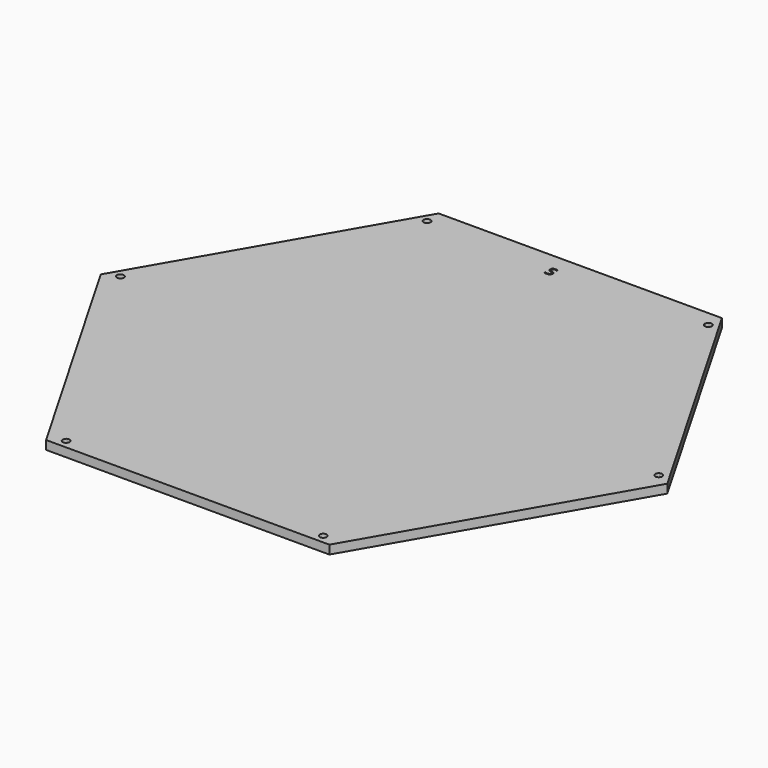
from build123d import *

# Parameters (mm, degrees)
F1_DEPTH     = 5
F3_DEPTH     = 25
F4_TEXT_SIZE = 8.1927412086
F5_DEPTH     = 25


# Not quite as in the source:
# - Text() gives the source's letters only with a copy of the font that has no kerning and outlines rounded to 1/6400 em; it was checked with that copy


with BuildPart() as f1:
    # F0 (on Top) → F1 (new body)
    with BuildSketch(Plane.XY):
        Polygon((-162, 140.2961154131), (-81, 0), (81, 0), (162, 140.2961154131), (81, 280.5922308262), (-81, 280.5922308262), align=None)
    extrude(amount=F1_DEPTH)

    # F2 (on face) → F3 (cut)
    with BuildSketch(Plane.XY.offset(5)):
        with BuildLine():
            Line((-78.4226497308, 271.5922308262), (-80.4226497308, 271.5922308262))
            Line((-80.4226497308, 271.5922308262), (-81.4226497308, 269.8601800186))
            ThreePointArc((-81.4226497308, 269.8601800186), (-79.4226497308, 269.8601800186), (-78.4226497308, 271.5922308262))
        make_face()
        with BuildLine():
            Line((-79.4226497308, 273.3242816337), (-80.4226497308, 271.5922308262))
            Line((-80.4226497308, 271.5922308262), (-78.4226497308, 271.5922308262))
            ThreePointArc((-78.4226497308, 271.5922308262), (-78.6905989232, 272.5922308262), (-79.4226497308, 273.3242816337))
        make_face()
        with BuildLine():
            Line((-81.4226497308, 269.8601800186), (-80.4226497308, 271.5922308262))
            Line((-80.4226497308, 271.5922308262), (-79.4226497308, 273.3242816337))
            ThreePointArc((-79.4226497308, 273.3242816337), (-82.1547005384, 272.5922308262), (-81.4226497308, 269.8601800186))
        make_face()
        with BuildLine():
            Line((79.4226497308, 273.3242816337), (80.4226497308, 271.5922308262))
            Line((80.4226497308, 271.5922308262), (81.4226497308, 269.8601800186))
            ThreePointArc((81.4226497308, 269.8601800186), (82.1547005384, 270.5922308262), (82.4226497308, 271.5922308262))
            ThreePointArc((82.4226497308, 271.5922308262), (81.4226497308, 273.3242816337), (79.4226497308, 273.3242816337))
        make_face()
        with BuildLine():
            ThreePointArc((79.4226497308, 273.3242816337), (78.6905989232, 272.5922308262), (78.4226497308, 271.5922308262))
            Line((78.4226497308, 271.5922308262), (80.4226497308, 271.5922308262))
            Line((80.4226497308, 271.5922308262), (79.4226497308, 273.3242816337))
        make_face()
        with BuildLine():
            Line((80.4226497308, 271.5922308262), (78.4226497308, 271.5922308262))
            ThreePointArc((78.4226497308, 271.5922308262), (79.4226497308, 269.8601800186), (81.4226497308, 269.8601800186))
            Line((81.4226497308, 269.8601800186), (80.4226497308, 271.5922308262))
        make_face()
        with BuildLine():
            ThreePointArc((155.9170962313, 144.2961154131), (154.9170962313, 146.0281662206), (152.9170962313, 146.0281662206))
            Line((152.9170962313, 146.0281662206), (153.9170962313, 144.2961154131))
            Line((153.9170962313, 144.2961154131), (154.9170962313, 142.5640646055))
            ThreePointArc((154.9170962313, 142.5640646055), (155.6491470389, 143.2961154131), (155.9170962313, 144.2961154131))
        make_face()
        with BuildLine():
            Line((154.9170962313, 142.5640646055), (153.9170962313, 144.2961154131))
            Line((153.9170962313, 144.2961154131), (152.9170962313, 142.5640646055))
            ThreePointArc((152.9170962313, 142.5640646055), (153.9170962313, 142.2961154131), (154.9170962313, 142.5640646055))
        make_face()
        with BuildLine():
            Line((153.9170962313, 144.2961154131), (152.9170962313, 146.0281662206))
            ThreePointArc((152.9170962313, 146.0281662206), (151.9170962313, 144.2961154131), (152.9170962313, 142.5640646055))
            Line((152.9170962313, 142.5640646055), (153.9170962313, 144.2961154131))
        make_face()
        with BuildLine():
            Line((73.494446436, 4.9999998882), (74.494446436, 6.7320506958))
            ThreePointArc((74.494446436, 6.7320506958), (72.494446436, 6.7320506958), (71.494446436, 4.9999998882))
            Line((71.494446436, 4.9999998882), (73.494446436, 4.9999998882))
        make_face()
        with BuildLine():
            ThreePointArc((75.494446436, 4.9999998882), (75.2264972436, 5.9999998882), (74.494446436, 6.7320506958))
            Line((74.494446436, 6.7320506958), (73.494446436, 4.9999998882))
            Line((73.494446436, 4.9999998882), (75.494446436, 4.9999998882))
        make_face()
        with BuildLine():
            Line((75.494446436, 4.9999998882), (73.494446436, 4.9999998882))
            Line((73.494446436, 4.9999998882), (71.494446436, 4.9999998882))
            ThreePointArc((71.494446436, 4.9999998882), (73.494446436, 2.9999998882), (75.494446436, 4.9999998882))
        make_face()
        with BuildLine():
            ThreePointArc((-71.494446436, 4.9999998882), (-72.494446436, 6.7320506958), (-74.494446436, 6.7320506958))
            Line((-74.494446436, 6.7320506958), (-73.494446436, 4.9999998882))
            Line((-73.494446436, 4.9999998882), (-71.494446436, 4.9999998882))
        make_face()
        with BuildLine():
            Line((-73.494446436, 4.9999998882), (-74.494446436, 6.7320506958))
            ThreePointArc((-74.494446436, 6.7320506958), (-75.2264972436, 5.9999998882), (-75.494446436, 4.9999998882))
            Line((-75.494446436, 4.9999998882), (-73.494446436, 4.9999998882))
        make_face()
        with BuildLine():
            Line((-71.494446436, 4.9999998882), (-73.494446436, 4.9999998882))
            Line((-73.494446436, 4.9999998882), (-75.494446436, 4.9999998882))
            ThreePointArc((-75.494446436, 4.9999998882), (-73.494446436, 2.9999998882), (-71.494446436, 4.9999998882))
        make_face()
        with BuildLine():
            ThreePointArc((-151.9170962313, 144.2961154131), (-152.1850454238, 145.2961154131), (-152.9170962313, 146.0281662206))
            Line((-152.9170962313, 146.0281662206), (-153.9170962313, 144.2961154131))
            Line((-153.9170962313, 144.2961154131), (-152.9170962313, 142.5640646055))
            ThreePointArc((-152.9170962313, 142.5640646055), (-152.1850454238, 143.2961154131), (-151.9170962313, 144.2961154131))
        make_face()
        with BuildLine():
            Line((-153.9170962313, 144.2961154131), (-152.9170962313, 146.0281662206))
            ThreePointArc((-152.9170962313, 146.0281662206), (-155.6491470389, 145.2961154131), (-154.9170962313, 142.5640646055))
            Line((-154.9170962313, 142.5640646055), (-153.9170962313, 144.2961154131))
        make_face()
        with BuildLine():
            Line((-152.9170962313, 142.5640646055), (-153.9170962313, 144.2961154131))
            Line((-153.9170962313, 144.2961154131), (-154.9170962313, 142.5640646055))
            ThreePointArc((-154.9170962313, 142.5640646055), (-153.9170962313, 142.2961154131), (-152.9170962313, 142.5640646055))
        make_face()
    extrude(amount=-F3_DEPTH, mode=Mode.SUBTRACT)

    # F4 (on face) → F5 (cut)
    with BuildSketch(Plane.XY.offset(5)):
        with Locations((-8.8470000774, 265.1734054089)):
            Text('S', F4_TEXT_SIZE, font='Open Sans', text_align=(TextAlign.LEFT, TextAlign.BOTTOM))
    extrude(amount=-F5_DEPTH, mode=Mode.SUBTRACT)


solid = f1.part
